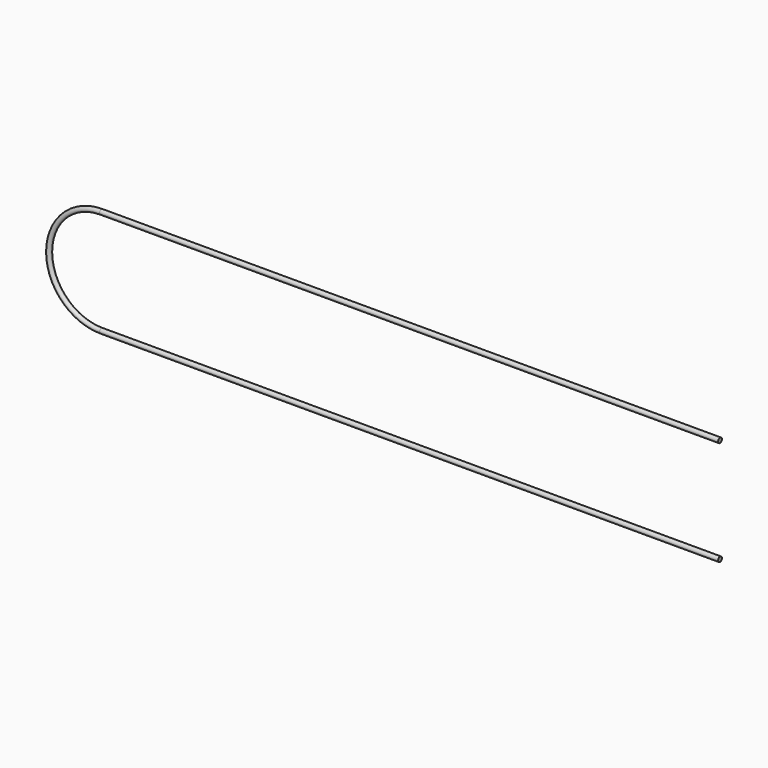
from build123d import *

# Parameters (mm, degrees)
F2_R = 0.5


# Not quite as in the source:
# - a feature of the source that left no trace in its solid (it failed there, or was rolled back) is left out


with BuildPart() as f3:
    # F3: sweep along a path in F1
    with BuildLine(Plane.XZ) as f3_path:
        Line((130, -11), (0, -11))
        ThreePointArc((0, -11), (-11, 0), (0, 11))
        Line((0, 11), (130, 11))
    # F2 (on Right) → F3 (sweep)
    with BuildSketch(Plane.YZ):
        with Locations((0, -11)):
            Circle(F2_R)
    sweep(path=f3_path.line)


solid = f3.part
